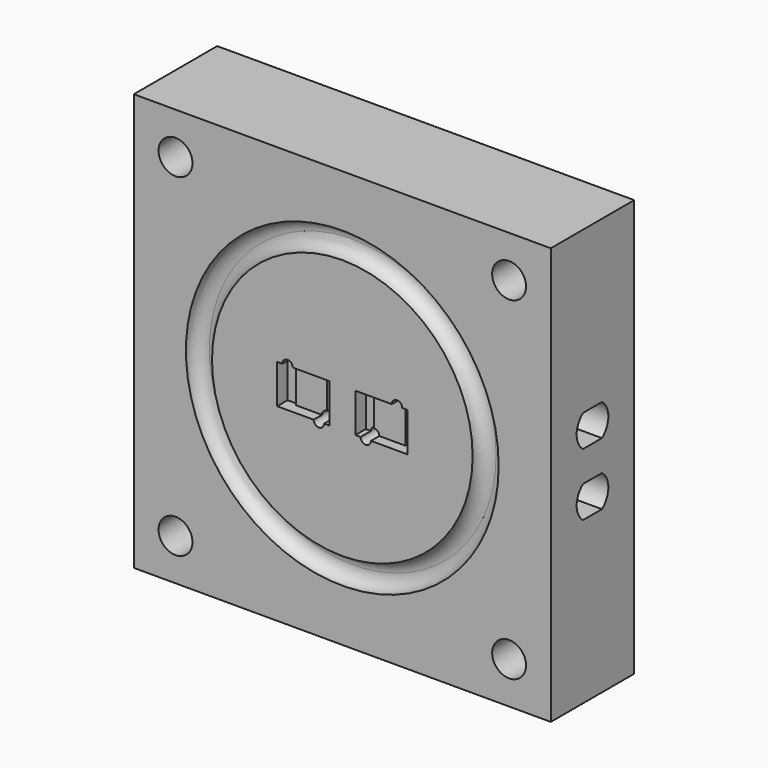
from build123d import *

# Parameters (mm, degrees)
F1_W      = 80
F1_H      = 80
F2_DEPTH  = 20
F4_R      = 3.25
F5_DEPTH  = 20.001
F4_R_2    = 30
F4_R_3    = 25
F6_DEPTH  = 2.5
F7_R      = 2.49999
F4_W      = 2
F4_H      = 3.75
F9_DEPTH  = 2.5
F10_DEPTH = 10
F12_DEPTH = 80.001
F13_DEPTH = 80.0010001
F14_DEPTH = 2


# Not quite as in the source:
# - two fillets or chamfers of one size are made in one step
# - a fillet or chamfer is up to 0.001 mm smaller than in the source, because OpenCascade refuses the exact size


with BuildPart() as f2:
    # F1 (on Front) → F2 (new body)
    with BuildSketch(Plane.XZ):
        with Locations((40, 40)):
            Rectangle(F1_W, F1_H)
    extrude(amount=F2_DEPTH)

    # F4 (on face) → F5 (cut, through all)
    with BuildSketch(Plane.XZ.offset(20)):
        with Locations((72, 8)):
            Circle(F4_R)
        with Locations((8, 8)):
            Circle(F4_R)
        with Locations((8, 72)):
            Circle(F4_R)
        with Locations((72, 72)):
            Circle(F4_R)
    extrude(amount=-F5_DEPTH, mode=Mode.SUBTRACT)

    # F4 (on face) → F6 (cut)
    with BuildSketch(Plane.XZ.offset(20)):
        with Locations((40, 40)):
            Circle(F4_R_2)
        with Locations((40, 40)):
            Circle(F4_R_3, mode=Mode.SUBTRACT)
    extrude(amount=-F6_DEPTH, mode=Mode.SUBTRACT)

    # F7 (radius 2.5 in the source; OpenCascade refuses exactly that, so slightly less here)
    f7_edges = [f2.edges().sort_by_distance(p)[0] for p in [
        (15, -17.5, 40),
        (10, -17.5, 40),
    ]]
    fillet(f7_edges, radius=F7_R)

    # F4 (on face) → F9 (cut)
    with BuildSketch(Plane.XZ.offset(20)):
        with BuildLine():
            Line((28.5, 43.75), (27.5, 43.75))
            Line((27.5, 43.75), (27.5, 40))
            Line((27.5, 40), (29.5, 40))
            Line((29.5, 40), (29.5, 42.75))
            ThreePointArc((29.5, 42.75), (28.7928932188, 43.0428932188), (28.5, 43.75))
        make_face()
        with Locations((28.5, 38.125)):
            Rectangle(F4_W, F4_H)
        with BuildLine():
            ThreePointArc((30.5, 43.75), (29.5, 44.75), (28.5, 43.75))
            Line((28.5, 43.75), (29.5, 43.75))
            Line((29.5, 43.75), (30.5, 43.75))
        make_face()
        with BuildLine():
            Line((52.5, 40), (52.5, 43.75))
            Line((52.5, 43.75), (51.5, 43.75))
            ThreePointArc((51.5, 43.75), (51.2071067812, 43.0428932188), (50.5, 42.75))
            Line((50.5, 42.75), (50.5, 40))
            Line((50.5, 40), (52.5, 40))
        make_face()
        with BuildLine():
            Line((37.5, 36.25), (37.5, 40))
            Line((37.5, 40), (35.5, 40))
            Line((35.5, 40), (35.5, 37.25))
            ThreePointArc((35.5, 37.25), (36.2071067812, 36.9571067812), (36.5, 36.25))
            Line((36.5, 36.25), (37.5, 36.25))
        make_face()
        with Locations((36.5, 41.875)):
            Rectangle(F4_W, F4_H)
        with Locations((43.5, 41.875)):
            Rectangle(F4_W, F4_H)
        with BuildLine():
            Line((44.5, 40), (42.5, 40))
            Line((42.5, 40), (42.5, 36.25))
            Line((42.5, 36.25), (43.5, 36.25))
            ThreePointArc((43.5, 36.25), (43.7928932188, 36.9571067812), (44.5, 37.25))
            Line((44.5, 37.25), (44.5, 40))
        make_face()
        with Locations((51.5, 38.125)):
            Rectangle(F4_W, F4_H)
        with BuildLine():
            Line((50.5, 43.75), (51.5, 43.75))
            ThreePointArc((51.5, 43.75), (50.5, 44.75), (49.5, 43.75))
            Line((49.5, 43.75), (50.5, 43.75))
        make_face()
        with BuildLine():
            ThreePointArc((36.5, 36.25), (36.2071067812, 36.9571067812), (35.5, 37.25))
            Line((35.5, 37.25), (35.5, 36.25))
            Line((35.5, 36.25), (36.5, 36.25))
        make_face()
        with BuildLine():
            Line((44.5, 36.25), (44.5, 37.25))
            ThreePointArc((44.5, 37.25), (43.7928932188, 36.9571067812), (43.5, 36.25))
            Line((43.5, 36.25), (44.5, 36.25))
        make_face()
    extrude(amount=-F9_DEPTH, mode=Mode.SUBTRACT)

    # F4 (on face) → F10 (cut)
    with BuildSketch(Plane.XZ.offset(20)):
        with BuildLine():
            ThreePointArc((30.5, 43.75), (29.5, 44.75), (28.5, 43.75))
            Line((28.5, 43.75), (29.5, 43.75))
            Line((29.5, 43.75), (30.5, 43.75))
        make_face()
        with BuildLine():
            Line((29.5, 43.75), (28.5, 43.75))
            ThreePointArc((28.5, 43.75), (28.7928932188, 43.0428932188), (29.5, 42.75))
            Line((29.5, 42.75), (29.5, 43.75))
        make_face()
        with BuildLine():
            Line((30.5, 43.75), (29.5, 43.75))
            Line((29.5, 43.75), (29.5, 42.75))
            ThreePointArc((29.5, 42.75), (30.2071067812, 43.0428932188), (30.5, 43.75))
        make_face()
        with BuildLine():
            Line((35.5, 36.25), (35.5, 37.25))
            ThreePointArc((35.5, 37.25), (34.7928932188, 36.9571067812), (34.5, 36.25))
            Line((34.5, 36.25), (35.5, 36.25))
        make_face()
        with BuildLine():
            ThreePointArc((36.5, 36.25), (36.2071067812, 36.9571067812), (35.5, 37.25))
            Line((35.5, 37.25), (35.5, 36.25))
            Line((35.5, 36.25), (36.5, 36.25))
        make_face()
        with BuildLine():
            ThreePointArc((34.5, 36.25), (35.5, 35.25), (36.5, 36.25))
            Line((36.5, 36.25), (35.5, 36.25))
            Line((35.5, 36.25), (34.5, 36.25))
        make_face()
        with BuildLine():
            Line((44.5, 36.25), (44.5, 37.25))
            ThreePointArc((44.5, 37.25), (43.7928932188, 36.9571067812), (43.5, 36.25))
            Line((43.5, 36.25), (44.5, 36.25))
        make_face()
        with BuildLine():
            ThreePointArc((45.5, 36.25), (45.2071067812, 36.9571067812), (44.5, 37.25))
            Line((44.5, 37.25), (44.5, 36.25))
            Line((44.5, 36.25), (45.5, 36.25))
        make_face()
        with BuildLine():
            Line((44.5, 36.25), (43.5, 36.25))
            ThreePointArc((43.5, 36.25), (44.5, 35.25), (45.5, 36.25))
            Line((45.5, 36.25), (44.5, 36.25))
        make_face()
        with BuildLine():
            Line((50.5, 43.75), (51.5, 43.75))
            ThreePointArc((51.5, 43.75), (50.5, 44.75), (49.5, 43.75))
            Line((49.5, 43.75), (50.5, 43.75))
        make_face()
        with BuildLine():
            Line((50.5, 42.75), (50.5, 43.75))
            Line((50.5, 43.75), (49.5, 43.75))
            ThreePointArc((49.5, 43.75), (49.7928932188, 43.0428932188), (50.5, 42.75))
        make_face()
        with BuildLine():
            ThreePointArc((50.5, 42.75), (51.2071067812, 43.0428932188), (51.5, 43.75))
            Line((51.5, 43.75), (50.5, 43.75))
            Line((50.5, 43.75), (50.5, 42.75))
        make_face()
    extrude(amount=-F10_DEPTH, mode=Mode.SUBTRACT)

    # F11 (on face) → F12 (cut, through all)
    with BuildSketch(Plane(origin=(0, 0, 0), x_dir=(0, -1, 0), z_dir=(-1, 0, 0))):
        with BuildLine():
            ThreePointArc((12.2666053913, 42.95), (13.3950773546, 44.293116947), (13.8, 46))
            ThreePointArc((13.8, 46), (13.3950773546, 47.706883053), (12.2666053913, 49.05))
            Line((12.2666053913, 49.05), (7.7333946087, 49.05))
            ThreePointArc((7.7333946087, 49.05), (6.2, 46), (7.7333946087, 42.95))
            Line((7.7333946087, 42.95), (12.2666053913, 42.95))
        make_face()
    extrude(amount=-F12_DEPTH, mode=Mode.SUBTRACT)

    # F11 (on face) → F13 (cut, through all)
    with BuildSketch(Plane(origin=(0, 0, 0), x_dir=(0, -1, 0), z_dir=(-1, 0, 0))):
        with BuildLine():
            ThreePointArc((12.2666053913, 42.95), (13.3950773546, 44.293116947), (13.8, 46))
            ThreePointArc((13.8, 46), (13.3950773546, 47.706883053), (12.2666053913, 49.05))
            Line((12.2666053913, 49.05), (7.7333946087, 49.05))
            ThreePointArc((7.7333946087, 49.05), (6.2, 46), (7.7333946087, 42.95))
            Line((7.7333946087, 42.95), (12.2666053913, 42.95))
        make_face()
        with BuildLine():
            ThreePointArc((12.2666053913, 30.95), (13.3950773546, 32.293116947), (13.8, 34))
            ThreePointArc((13.8, 34), (13.3950773546, 35.706883053), (12.2666053913, 37.05))
            Line((12.2666053913, 37.05), (7.7333946087, 37.05))
            ThreePointArc((7.7333946087, 37.05), (6.2, 34), (7.7333946087, 30.95))
            Line((7.7333946087, 30.95), (12.2666053913, 30.95))
        make_face()
    extrude(amount=-F13_DEPTH, mode=Mode.SUBTRACT)

    # F4 (on face) → F14 (cut)
    with BuildSketch(Plane.XZ.offset(20)):
        with BuildLine():
            Line((29.5, 42.75), (29.5, 40))
            Line((29.5, 40), (35.5, 40))
            Line((35.5, 40), (35.5, 43.75))
            Line((35.5, 43.75), (30.5, 43.75))
            ThreePointArc((30.5, 43.75), (30.2071067812, 43.0428932188), (29.5, 42.75))
        make_face()
        with BuildLine():
            Line((35.5, 40), (29.5, 40))
            Line((29.5, 40), (29.5, 36.25))
            Line((29.5, 36.25), (34.5, 36.25))
            ThreePointArc((34.5, 36.25), (34.7928932188, 36.9571067812), (35.5, 37.25))
            Line((35.5, 37.25), (35.5, 40))
        make_face()
        with BuildLine():
            Line((44.5, 43.75), (44.5, 40))
            Line((44.5, 40), (50.5, 40))
            Line((50.5, 40), (50.5, 42.75))
            ThreePointArc((50.5, 42.75), (49.7928932188, 43.0428932188), (49.5, 43.75))
            Line((49.5, 43.75), (44.5, 43.75))
        make_face()
        with BuildLine():
            Line((50.5, 40), (44.5, 40))
            Line((44.5, 40), (44.5, 37.25))
            ThreePointArc((44.5, 37.25), (45.2071067812, 36.9571067812), (45.5, 36.25))
            Line((45.5, 36.25), (50.5, 36.25))
            Line((50.5, 36.25), (50.5, 40))
        make_face()
    extrude(amount=-F14_DEPTH, mode=Mode.SUBTRACT)


solid = f2.part
